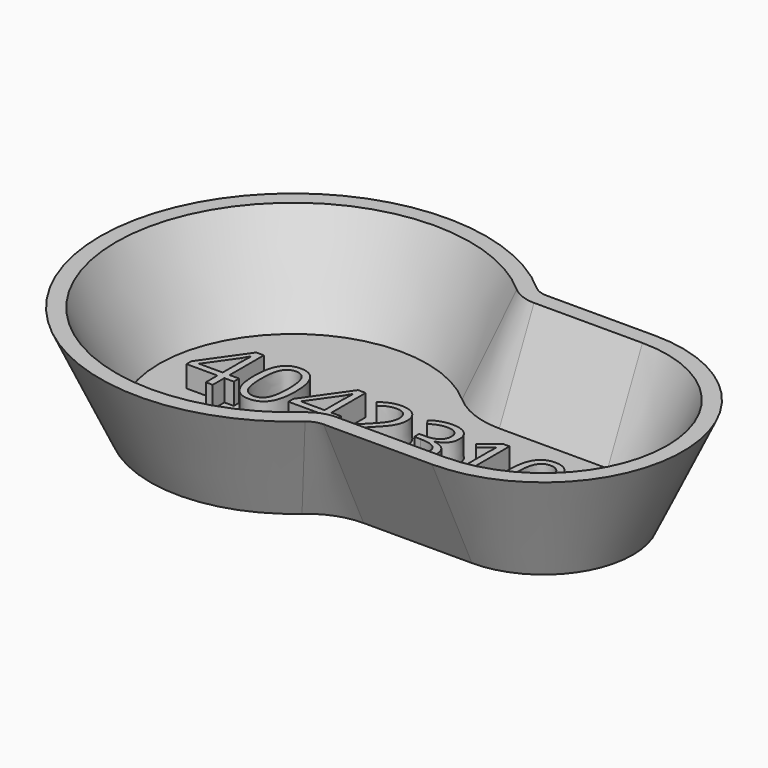
from build123d import *

# Parameters (mm, degrees)
F1_DEPTH     = 15
F1_TAPER     = -25
F2_T         = 2
F3_TEXT_SIZE = 12.4548864199
F4_DEPTH     = 3


# Not quite as in the source:
# - a shell that OpenCascade refuses in one call is made with other operations: the cavity is built on its own and cut out
# - Text() gives the source's letters only with a copy of the font that has no kerning and outlines rounded to 1/6400 em; it was checked with that copy


with BuildPart() as f1:
    # F0 (on Top) → F1 (new body)
    with BuildSketch(Plane.XY):
        with BuildLine():
            ThreePointArc((-0.156865167, 12.5), (-3.6923990729, 13.1458565331), (-6.7712434447, 15))
            ThreePointArc((-6.7712434447, 15), (-40, 0), (-6.7712434447, -15))
            ThreePointArc((-6.7712434447, -15), (-3.6923990729, -13.1458565331), (-0.156865167, -12.5))
            Line((-0.156865167, -12.5), (15, -12.5))
            ThreePointArc((15, -12.5), (27.5, 0), (15, 12.5))
            Line((15, 12.5), (-0.156865167, 12.5))
        make_face()
    extrude(amount=F1_DEPTH, taper=F1_TAPER)

    # F2: shell of thickness 2, made by hand


with BuildPart() as f2_core1:
    # F2_t2: copy of F1
    add(f1.part)

    # the walls: a layer under each face that stays
    f2_faces = [f2_core1.faces().sort_by_distance(p)[0] for p in [
        (7.4215674165, 15.9973074362, 7.5),
        (-2.4559141709, 16.4172880836, 7.5),
        (-43.4973074362, 0, 7.5),
        (-2.4559141709, -16.4172880836, 7.5),
        (7.4215674165, -15.9973074362, 7.5),
        (30.9973074362, 0, 7.5),
        (-6.25, 0, 0),
    ]]
    thicken(f2_faces, amount=-F2_T, mode=Mode.SUBTRACT)


with BuildPart() as f1_1:
    add(f1.part)

    # what is left inside the walls is the cavity
    f2_cavity = [f2_core1.part.solids().sort_by_distance(p)[0] for p in [
        (6.595953, 0, 14.98),
    ]]
    add(f2_cavity, mode=Mode.SUBTRACT)

    # F3 (on face) → F4 (join)
    with BuildSketch(Plane.XY.offset(2)):
        with Locations((-33, -4.7677234526)):
            Text('40423101', F3_TEXT_SIZE, font='Open Sans', text_align=(TextAlign.LEFT, TextAlign.BOTTOM))
    extrude(amount=F4_DEPTH)


solid = f1_1.part
